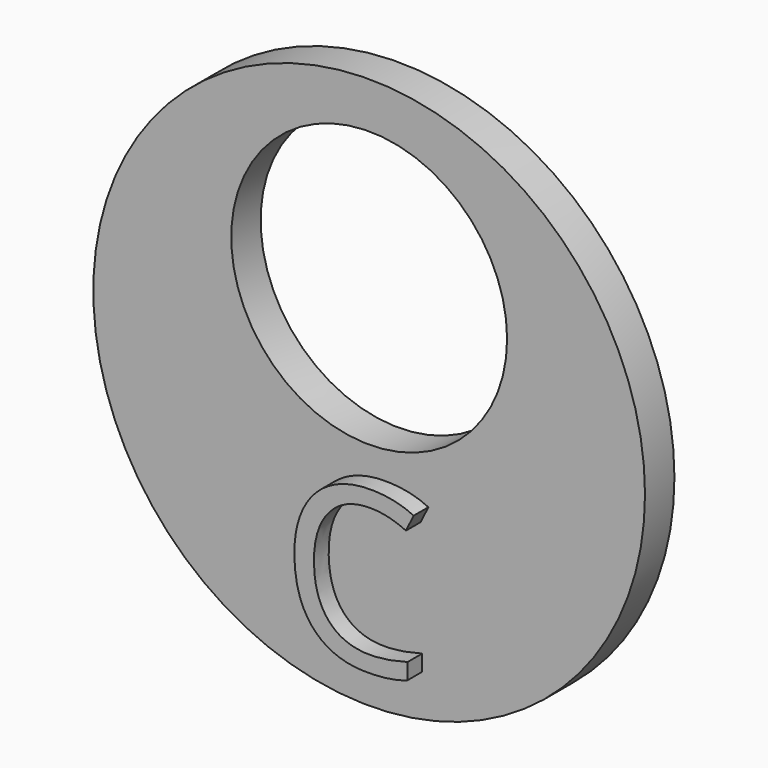
from build123d import *

# Parameters (mm, degrees)
F0_R         = 15
F0_R_2       = 7.5
F1_DEPTH     = 2
F2_TEXT_SIZE = 12.0131393712
F3_DEPTH     = 1


# Not quite as in the source:
# - Text() gives the source's letters only with a copy of the font that has no kerning and outlines rounded to 1/6400 em; it was checked with that copy


with BuildPart() as f1:
    # F0 (on Front) → F1 (new body)
    with BuildSketch(Plane.XZ):
        Circle(F0_R)
        with Locations((0, 5)):
            Circle(F0_R_2, mode=Mode.SUBTRACT)
    extrude(amount=F1_DEPTH)

    # F2 (on face) → F3 (join)
    with BuildSketch(Plane.XZ.offset(2)):
        with Locations((-4, -12.6494603473)):
            Text('C', F2_TEXT_SIZE, font='Open Sans', text_align=(TextAlign.LEFT, TextAlign.BOTTOM))
    extrude(amount=F3_DEPTH)


solid = f1.part
